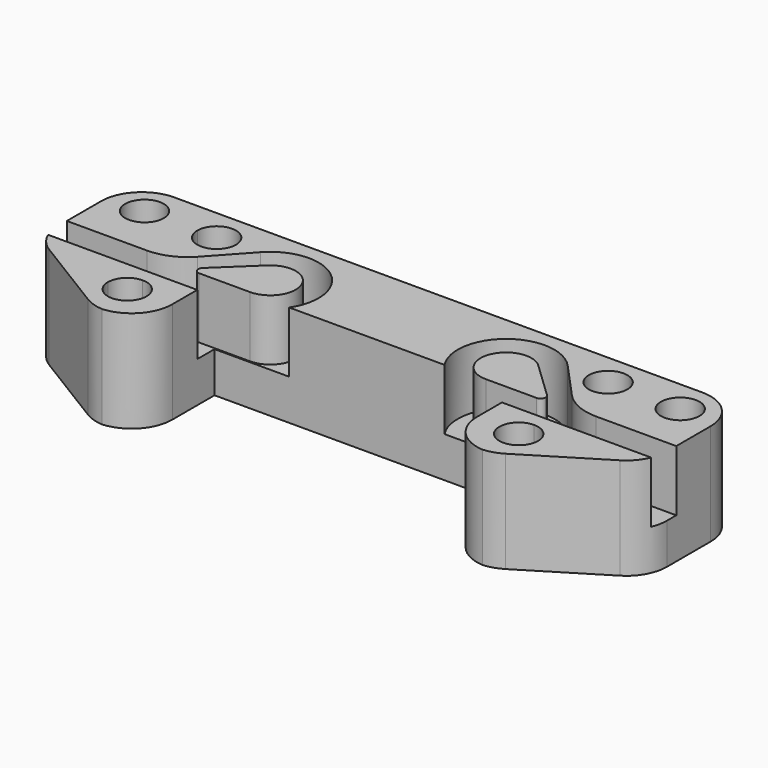
from build123d import *

# Parameters (mm, degrees)
F1_DEPTH    = 10
F2_W        = 10.0960650777
F2_H        = 2.7
F3_DEPTH    = 6
F4_R        = 5
F5_T1_DEPTH = 21.1923143391
F5_T3_DEPTH = 15.6473434867
F5_T5_DEPTH = 30
F7_DEPTH    = 2


# Not quite as in the source:
# - a fillet or chamfer that OpenCascade refuses, or shapes differently, is made with other operations: its cross-section is extruded or revolved along the edge and cut away or added


with BuildPart() as f1:
    # F0 (on Top) → F1 (new body)
    with BuildSketch(Plane.XY):
        Polygon((30, 9), (0, 9), (0, -1.8), (15, -1.8), (15, -9), (19.5954625243, -9), (30, -2.6151265483), align=None)
        with BuildLine():
            ThreePointArc((21.17, -5.2), (17.9264971157, -6.5435028843), (19.27, -3.3))
            ThreePointArc((19.27, -3.3), (20.6135028843, -3.8564971157), (21.17, -5.2))
        make_face(mode=Mode.SUBTRACT)
        with BuildLine():
            ThreePointArc((19.27, 3.9), (17.9264971157, 7.1435028843), (21.17, 5.8))
            ThreePointArc((21.17, 5.8), (20.6135028843, 4.4564971157), (19.27, 3.9))
        make_face(mode=Mode.SUBTRACT)
        with BuildLine():
            ThreePointArc((24.47, 5.8), (26.37, 7.7), (28.27, 5.8))
            ThreePointArc((28.27, 5.8), (26.37, 3.9), (24.47, 5.8))
        make_face(mode=Mode.SUBTRACT)
    extrude(amount=F1_DEPTH)

    # F2 (on face) → F3 (cut)
    with BuildSketch(Plane.XY.offset(10)):
        with BuildLine():
            ThreePointArc((11.6039349223, 0.3250306588), (9.2827431951, 3.7535073497), (13.3280728534, 4.6353754864))
            Line((13.3280728534, 4.6353754864), (16.2527744297, 1.8499454137))
            ThreePointArc((16.2527744297, 1.8499454137), (16.328577113, 2.3348713274), (16.3539349223, 2.8250306588))
            ThreePointArc((16.3539349223, 2.8250306588), (16.0328522645, 4.5417691876), (15.1130123218, 6.0264172029))
            ThreePointArc((15.1130123218, 6.0264172029), (7.5069370658, 5.2285923001), (10.5215341623, -1.8))
            Line((10.5215341623, -1.8), (12.6863356823, -1.8))
            ThreePointArc((12.6863356823, -1.8), (14.376262754, -1.0320016711), (15.6428085277, 0.3250306588))
            Line((15.6428085277, 0.3250306588), (11.6039349223, 0.3250306588))
        make_face()
        with BuildLine():
            ThreePointArc((16.3539349223, 2.8250306588), (16.328577113, 2.3348713274), (16.2527744297, 1.8499454137))
            Line((16.2527744297, 1.8499454137), (16.9487625085, 1.1870996243))
            ThreePointArc((16.9487625085, 1.1870996243), (17.0635074373, 1.0219903081), (17.1039349223, 0.8250306588))
            ThreePointArc((17.1039349223, 0.8250306588), (16.9574883129, 0.4714772682), (16.6039349223, 0.3250306588))
            Line((16.6039349223, 0.3250306588), (15.6428085277, 0.3250306588))
            ThreePointArc((15.6428085277, 0.3250306588), (14.376262754, -1.0320016711), (12.6863356823, -1.8))
            Line((12.6863356823, -1.8), (15, -1.8))
            Line((15, -1.8), (15, -1.9249693412))
            Line((15, -1.9249693412), (19.9039349223, -1.9249693412))
            Line((19.9039349223, -1.9249693412), (19.9039349223, 0.7750306588))
            Line((19.9039349223, 0.7750306588), (15.1130123218, 6.0264172029))
            ThreePointArc((15.1130123218, 6.0264172029), (16.0328522645, 4.5417691876), (16.3539349223, 2.8250306588))
        make_face()
        with Locations((24.9519674612, -0.5749693412)):
            Rectangle(F2_W, F2_H)
    extrude(amount=-F3_DEPTH, mode=Mode.SUBTRACT)

    # F4
    f4_edges = [f1.edges().sort_by_distance(p)[0] for p in [
        (19.903935, 0.775031, 7),
    ]]
    fillet(f4_edges, radius=F4_R)

    # F5: fillet of radius 4 on 4 edges, made by hand

    # F5_s2 → F5_t1 (cut)
    with BuildSketch(Plane.XY.offset(-5.5961571696)):
        with BuildLine():
            ThreePointArc((30, -0.3766636805), (29.4905957559, -2.3300559271), (28.0921293656, -3.7859150232))
            Line((28.0921293656, -3.7859150232), (30, -2.6151265483))
            Line((30, -2.6151265483), (30, -0.3766636805))
        make_face()
    extrude(amount=F5_T1_DEPTH, mode=Mode.SUBTRACT)

    # F5_s4 → F5_t3 (cut)
    with BuildSketch(Plane.XY.offset(-2.8236717433)):
        with BuildLine():
            ThreePointArc((20.5581231925, -8.4092513427), (19.5529608525, -8.8494808332), (18.465993827, -9))
            Line((18.465993827, -9), (19.5954625243, -9))
            Line((19.5954625243, -9), (20.5581231925, -8.4092513427))
        make_face()
    extrude(amount=F5_T3_DEPTH, mode=Mode.SUBTRACT)

    # F5_s6 → F5_t5 (cut)
    with BuildSketch(Plane.XY.offset(-10)):
        with BuildLine():
            ThreePointArc((15, -5), (16.1715728753, -7.8284271247), (19, -9))
            Line((19, -9), (15, -9))
            Line((15, -9), (15, -5))
        make_face()
        with BuildLine():
            ThreePointArc((30, 5), (28.8284271247, 7.8284271247), (26, 9))
            Line((26, 9), (30, 9))
            Line((30, 9), (30, 5))
        make_face()
    extrude(amount=F5_T5_DEPTH, mode=Mode.SUBTRACT)

    # F6 (on face) → F7 (cut)
    with BuildSketch(Plane.XZ.offset(1.8)):
        Polygon((0, 10), (0, 0), (15, 0), (15, 4), (10.5215341623, 4), (10.5215341623, 10), align=None)
    extrude(amount=-F7_DEPTH, mode=Mode.SUBTRACT)

    # F8: F1 across plane


with BuildPart() as f1_1:
    add(f1.part)
    add(f1.part.mirror(Plane.YZ))


solid = f1_1.part
